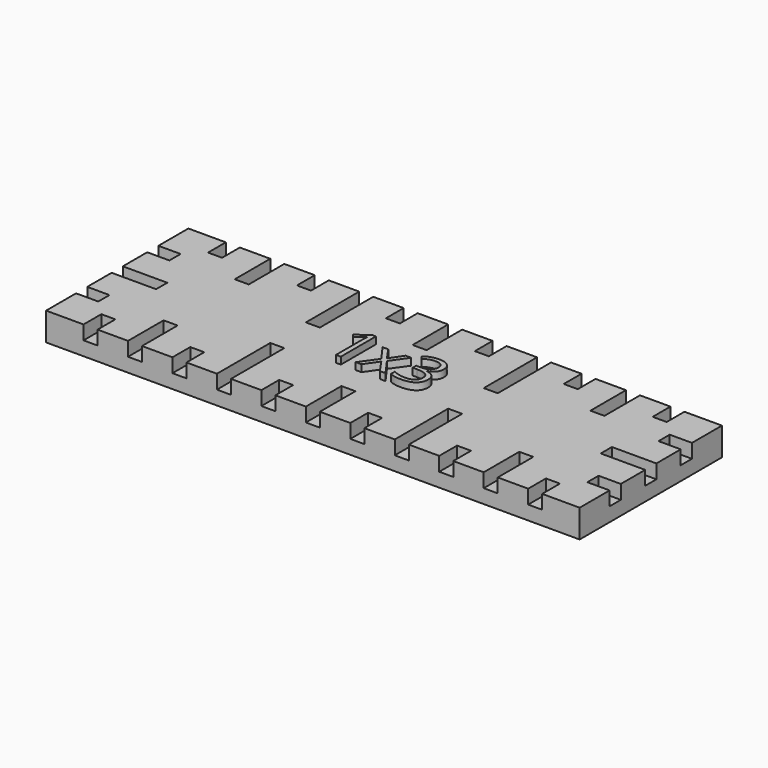
from build123d import *

# Parameters (mm, degrees)
F0_W         = 76.2
F0_H         = 25.4
F1_DEPTH     = 4
F2_W         = 2
F2_H         = 12.7
F2_H_2       = 6.35
F2_W_2       = 12.7
F2_H_3       = 2
F2_W_3       = 6.35
F2_H_4       = 19.05
F3_DEPTH     = 2
F4_TEXT_SIZE = 8.7834936047
F5_DEPTH     = 1


# Not quite as in the source:
# - Text() gives the source's letters only with a copy of the font that has no kerning and outlines rounded to 1/6400 em; it was checked with that copy


with BuildPart() as f1:
    # F0 (on Top) → F1 (new body)
    with BuildSketch(Plane.XY):
        Rectangle(F0_W, F0_H)
    extrude(amount=F1_DEPTH)

    # F2 (on face) → F3 (cut)
    with BuildSketch(Plane.XY.offset(4)):
        with Locations((0, -12.7)):
            Rectangle(F2_W, F2_H)
        with Locations((6.35, -12.7)):
            Rectangle(F2_W, F2_H_2)
        with Locations((-6.35, -12.7)):
            Rectangle(F2_W, F2_H_2)
        with Locations((-38.1, 0)):
            Rectangle(F2_W_2, F2_H_3)
        with Locations((-38.1, 6.35)):
            Rectangle(F2_W_3, F2_H_3)
        with Locations((-38.1, -6.35)):
            Rectangle(F2_W_3, F2_H_3)
        with Locations((0, 12.7)):
            Rectangle(F2_W, F2_H)
        with Locations((-6.35, 12.7)):
            Rectangle(F2_W, F2_H_2)
        with Locations((6.35, 12.7)):
            Rectangle(F2_W, F2_H_2)
        with Locations((38.1, 0)):
            Rectangle(F2_W_2, F2_H_3)
        with Locations((38.1, -6.35)):
            Rectangle(F2_W_3, F2_H_3)
        with Locations((38.1, 6.35)):
            Rectangle(F2_W_3, F2_H_3)
        with Locations((-12.7, 12.7000001177)):
            Rectangle(F2_W, F2_H_4)
        with Locations((-19.05, 12.7000001177)):
            Rectangle(F2_W, F2_H_2)
        with Locations((-12.7, -12.7000005066)):
            Rectangle(F2_W, F2_H_4)
        with Locations((-19.05, -12.7000005066)):
            Rectangle(F2_W, F2_H_2)
        with Locations((12.700000225, -12.7)):
            Rectangle(F2_W, F2_H_4)
        with Locations((19.050000225, -12.7)):
            Rectangle(F2_W, F2_H_2)
        with Locations((12.700000225, 12.7)):
            Rectangle(F2_W, F2_H_4)
        with Locations((19.050000225, 12.7)):
            Rectangle(F2_W, F2_H_2)
        with Locations((25.4000000715, 12.7)):
            Rectangle(F2_W, F2_H)
        with Locations((31.7500000715, 12.7)):
            Rectangle(F2_W, F2_H_2)
        with Locations((25.4000000715, -12.7)):
            Rectangle(F2_W, F2_H)
        with Locations((31.7500000715, -12.7)):
            Rectangle(F2_W, F2_H_2)
        with Locations((-25.4000000715, -12.7000005066)):
            Rectangle(F2_W, F2_H)
        with Locations((-31.7500000715, -12.7000005066)):
            Rectangle(F2_W, F2_H_2)
        with Locations((-25.4, 12.7000005066)):
            Rectangle(F2_W, F2_H)
        with Locations((-31.75, 12.7000005066)):
            Rectangle(F2_W, F2_H_2)
    extrude(amount=-F3_DEPTH, mode=Mode.SUBTRACT)

    # F4 (on face) → F5 (join)
    with BuildSketch(Plane.XY.offset(4)):
        with Locations((-7.35, -2.3543973291)):
            Text('1x3', F4_TEXT_SIZE, font='Open Sans', text_align=(TextAlign.LEFT, TextAlign.BOTTOM))
    extrude(amount=F5_DEPTH)


solid = f1.part
